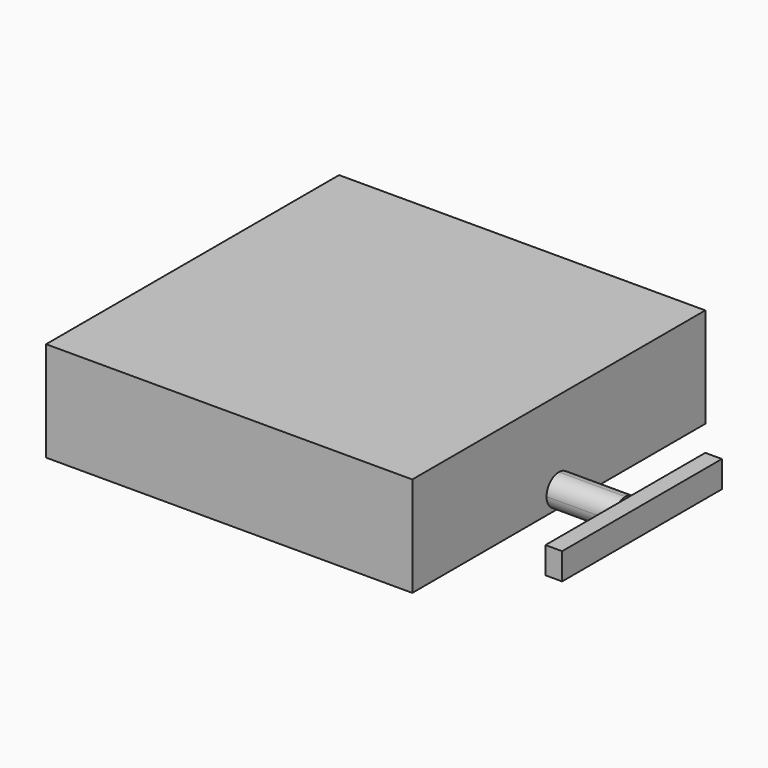
from build123d import *

# Parameters (mm, degrees)
F0_W     = 31.75
F0_H     = 31.75
F1_DEPTH = 1.5875
F0_W_2   = 6.35
F0_H_2   = 1.4605
F2_DEPTH = 1.4605
F3_R     = 1.46049
F5_DEPTH = 1.5875
F6_DEPTH = 6.35


# Not quite as in the source:
# - a fillet or chamfer is up to 0.001 mm smaller than in the source, because OpenCascade refuses the exact size
# - ends of sketch curves that miss each other by under 0.0002 mm in the source are joined


with BuildPart() as f1:
    # F0 (on Top) → F1 (new body, symmetric)
    with BuildSketch(Plane.XY):
        Polygon((17.4625, 17.4625), (-17.4625, 17.4625), (-17.4625, 1.4605), (-17.4625, 0), (-17.4625, -1.4605), (-17.4625, -17.4625), (17.4625, -17.4625), (17.4625, -1.4605), (17.4625, 0), (17.4625, 1.4605), align=None)
        Rectangle(F0_W, F0_H, mode=Mode.SUBTRACT)
        Rectangle(F0_W, F0_H)
    extrude(amount=F1_DEPTH, both=True)

    # F0 (on Top) → F2 (join, symmetric)
    with BuildSketch(Plane.XY):
        with Locations((-20.6375, 0.73025)):
            Rectangle(F0_W_2, F0_H_2)
        with Locations((-20.6375, -0.73025)):
            Rectangle(F0_W_2, F0_H_2)
        with Locations((20.6375, 0.73025)):
            Rectangle(F0_W_2, F0_H_2)
        with Locations((20.6375, -0.73025)):
            Rectangle(F0_W_2, F0_H_2)
    extrude(amount=F2_DEPTH, both=True)

    # F3 (radius 1.4605 in the source; OpenCascade refuses exactly that, so slightly less here)
    f3_edges = [f1.edges().sort_by_distance(p)[0] for p in [
        (-20.6375, -1.4605, 1.4605),
        (-20.6375, 1.4605, 1.4605),
        (-20.6375, -1.4605, -1.4605),
        (-20.6375, 1.4605, -1.4605),
        (20.6375, 1.4605, -1.4605),
        (20.6375, -1.4605, -1.4605),
        (20.6375, -1.4605, 1.4605),
        (20.6375, 1.4605, 1.4605),
    ]]
    fillet(f3_edges, radius=F3_R)

    # F4 (on face) → F5 (join)
    with BuildSketch(Plane.YZ.offset(23.8125)):
        with BuildLine():
            Line((9.525, 1.27), (0.7212287186, 1.27))
            ThreePointArc((0.7212287186, 1.27), (1.2622230895, 0.7347542799), (1.4605, 1e-05))
            ThreePointArc((1.4605, 1e-05), (1.2622230895, -0.7347542799), (0.7212287186, -1.27))
            Line((0.7212287186, -1.27), (9.525, -1.27))
            Line((9.525, -1.27), (9.525, 1.27))
        make_face()
        with BuildLine():
            Line((-0.7212287186, 1.27), (-9.525, 1.27))
            Line((-9.525, 1.27), (-9.525, -1.27))
            Line((-9.525, -1.27), (-0.7212287186, -1.27))
            ThreePointArc((-0.7212287186, -1.27), (-1.2622230895, -0.7347542799), (-1.4605, -1e-05))
            ThreePointArc((-1.4605, -1e-05), (-1.2622230895, 0.7347542799), (-0.7212287186, 1.27))
        make_face()
        with BuildLine():
            Line((0.7212287186, 1.27), (-0.7212287186, 1.27))
            ThreePointArc((-0.7212287186, 1.27), (-1.2622230895, 0.7347542799), (-1.4605, 1e-05))
            ThreePointArc((-1.4605, 1e-05), (-1.2622230895, -0.7347542799), (-0.7212287186, -1.27))
            Line((-0.7212287186, -1.27), (0.7212287186, -1.27))
            ThreePointArc((0.7212287186, -1.27), (1.2622230895, -0.7347542799), (1.4605, -1e-05))
            ThreePointArc((1.4605, -1e-05), (1.2622230895, 0.7347542799), (0.7212287186, 1.27))
        make_face()
    extrude(amount=F5_DEPTH)

    # F6 (add): a face of the model
    f6_faces = [f1.faces().sort_by_distance(p)[0] for p in [
        (0, 0, 1.5875),
    ]]
    extrude(f6_faces, amount=F6_DEPTH)


solid = f1.part
